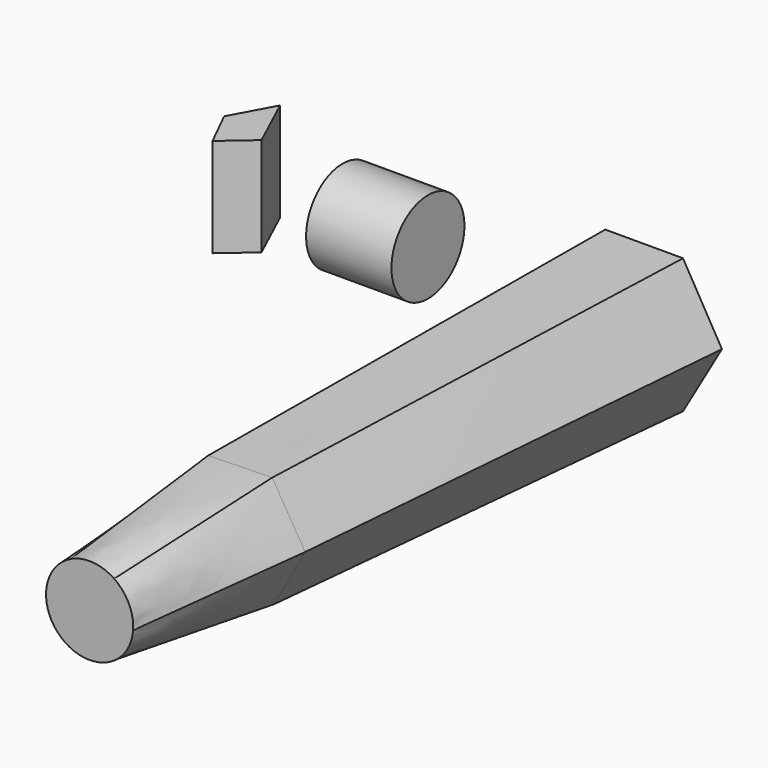
from build123d import *

# Parameters (mm, degrees)
F1_DEPTH = 52.07
F2_R     = 24.0348564639
F3_DEPTH = 44.958


# Not quite as in the source:
# - the arcs of a loft's sections are written as splines that run evenly, so that the points pair up as in the source's solid


with BuildPart() as f1:
    # F0 (on Top) → F1 (new body)
    with BuildSketch(Plane.XY):
        Polygon((-128.12936306, 0), (-118.1188970804, -20.1593339443), (-102.8770580888, -6.9779586047), (-116.2189766765, 21.9337996095), align=None)
    extrude(amount=F1_DEPTH)


with BuildPart() as f3:
    # F2 (on Right) → F3 (new body)
    with BuildSketch(Plane.YZ):
        with Locations((-25.9751360863, 43.7066555023)):
            Circle(F2_R)
    extrude(amount=-F3_DEPTH)


with BuildPart() as f7:
    # F4 (on Front) → F7 section 0
    with BuildSketch(Plane.XZ):
        Polygon((113.5863239066, 64.8323372006), (72.628227423, 64.8323372006), (52.1491791811, 29.3615851551), (72.628227423, -6.1091668904), (113.5863239066, -6.1091668904), (134.0653721485, 29.3615851551), align=None)
    # F6 (on offset) → F7 section 1
    with BuildSketch(Plane.XZ.offset(247.396)):
        Polygon((112.4704657081, 28.843481159), (95.0816841837, 57.6574466469), (61.4336673252, 57.0053028498), (45.1744319912, 27.5391935648), (62.5632135156, -1.274771923), (96.2112303741, -0.6226281259), align=None)
    loft()

    # F7_face (on face) → F10 section 0
    with BuildSketch(Plane(origin=(78.8224488497, -247.396, 28.1913373619), x_dir=(1, 0, 0), z_dir=(0, -1, 0))):
        Polygon((33.6480168585, 0.6521437971), (16.259235334, 29.4661092849), (-17.3887815244, 28.8139654879), (-33.6480168585, -0.6521437971), (-16.259235334, -29.4661092849), (17.3887815244, -28.8139654879), align=None)
    # F9 (on offset) → F10 section 1
    with BuildSketch(Plane.XZ.offset(342.392)):
        with BuildLine():
            add(Edge.make_bspline(
                [(87.8640765562, 47.0690177587), (85.6570363119, 48.5734477992), (83.1853326809, 49.6884427268), (78.0083630622, 51.0061419006), (75.3043706745, 51.2085219762), (69.9889308654, 50.6761262752), (67.3787911096, 49.9414814748), (64.9723963541, 48.7823435763)],
                knots=[0, 0, 0, 0, 0.3333333333, 0.3333333333, 0.6666666667, 0.6666666667, 1, 1, 1, 1], degree=3))
            add(Edge.make_bspline(
                [(64.9723963541, 48.7823435763), (62.5660015987, 47.6232056779), (60.3645358508, 46.0401450066), (56.6348900825, 42.2156073891), (55.1076276019, 39.9750713274), (52.9109758993, 35.1055675701), (52.2421270813, 32.4777978338), (52.0427725701, 29.8142298949)],
                knots=[0, 0, 0, 0, 0.3333333333, 0.3333333333, 0.6666666667, 0.6666666667, 1, 1, 1, 1], degree=3))
            add(Edge.make_bspline(
                [(52.0427725701, 29.8142298949), (51.843418059, 27.150661956), (52.1136559421, 24.4526063571), (53.5609797924, 19.3103695658), (54.7377096996, 16.8674534286), (57.856497806, 12.5303453722), (59.7977887439, 10.6372204364), (62.0048289881, 9.1327903958)],
                knots=[0, 0, 0, 0, 0.3333333333, 0.3333333333, 0.6666666667, 0.6666666667, 1, 1, 1, 1], degree=3))
            add(Edge.make_bspline(
                [(62.0048289881, 9.1327903958), (64.2118692324, 7.6283603553), (66.6835728634, 6.5133654277), (71.8605424821, 5.195666254), (74.5645348698, 4.9932861784), (79.8799746788, 5.5256818794), (82.4901144347, 6.2603266798), (84.8965091901, 7.4194645782)],
                knots=[0, 0, 0, 0, 0.3333333333, 0.3333333333, 0.6666666667, 0.6666666667, 1, 1, 1, 1], degree=3))
            add(Edge.make_bspline(
                [(84.8965091901, 7.4194645782), (87.3029039455, 8.5786024767), (89.5043696934, 10.1616631479), (93.2340154618, 13.9862007655), (94.7612779424, 16.2267368271), (96.957929645, 21.0962405845), (97.626778463, 23.7240103208), (97.8261329741, 26.3875782597)],
                knots=[0, 0, 0, 0, 0.3333333333, 0.3333333333, 0.6666666667, 0.6666666667, 1, 1, 1, 1], degree=3))
            add(Edge.make_bspline(
                [(97.8261329741, 26.3875782597), (98.0254874853, 29.0511461986), (97.7552496022, 31.7492017975), (96.3079257519, 36.8914385888), (95.1311958447, 39.334354726), (92.0124077383, 43.6714627824), (90.0711168004, 45.5645877182), (87.8640765562, 47.0690177587)],
                knots=[0, 0, 0, 0, 0.3333333333, 0.3333333333, 0.6666666667, 0.6666666667, 1, 1, 1, 1], degree=3))
        make_face()
    loft(ruled=True)


solid = Compound([f1.part, f3.part, f7.part])
